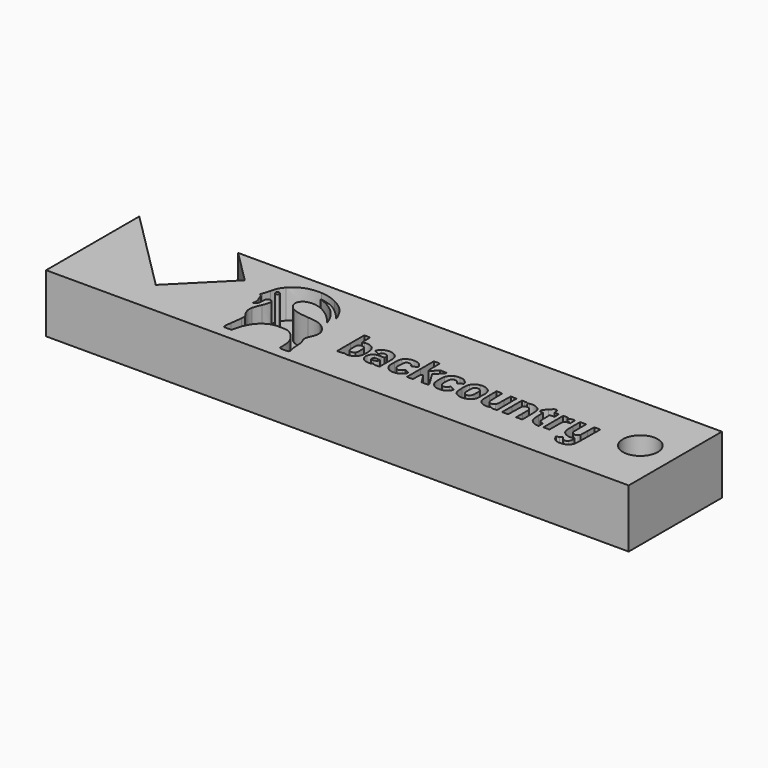
from build123d import *

# Parameters (mm, degrees)
F0_R     = 1.905
F1_DEPTH = 3.175
F3_DEPTH = 25.4


# Not quite as in the source:
# - ends of sketch curves that miss each other by under 0.0002 mm in the source are joined


with BuildPart() as f1:
    # F0 (on Top) → F1 (new body, symmetric)
    with BuildSketch(Plane.XY):
        Polygon((-31.75, -6.35), (31.75, -6.35), (31.75, 6.35), (-20.9736926547, 6.35), (-17.3815902063, 2.7578975516), (-22.7697438789, -2.6302561211), (-31.75, 6.35), align=None)
        with Locations((27.94, 0)):
            Circle(F0_R, mode=Mode.SUBTRACT)
    extrude(amount=F1_DEPTH, both=True)

    # F2 (on Top) → F3 (cut)
    with BuildSketch(Plane.XY):
        with BuildLine():
            add(Edge.make_bspline(
                [(-7.2094861414, -5.1238648126), (-7.2844689878, -5.0802139859), (-7.2989422964, -4.9953436696), (-7.2989422964, -4.5994253193)],
                knots=[0, 0, 0, 0, 1, 1, 1, 1], degree=3))
            add(Edge.make_bspline(
                [(-6.7301263581, -5.1775256832), (-6.9445733291, -5.1767519197), (-7.1602848509, -5.1525291904), (-7.2094861414, -5.1238648126)],
                knots=[0, 0, 0, 0, 1, 1, 1, 1], degree=3))
            add(Edge.make_bspline(
                [(-6.2994829734, -4.731018672), (-6.1786161943, -5.1344968151), (-6.2220690357, -5.1795470484), (-6.7301263581, -5.1775256832)],
                knots=[0, 0, 0, 0, 1, 1, 1, 1], degree=3))
            add(Edge.make_bspline(
                [(-6.4145096801, -3.7988983941), (-6.39840066, -4.1771751812), (-6.3514717779, -4.5574775093), (-6.2994829734, -4.731018672)],
                knots=[0, 0, 0, 0, 1, 1, 1, 1], degree=3))
            add(Edge.make_bspline(
                [(-6.5358053454, -2.9810219707), (-6.4648588427, -3.115930716), (-6.4350259592, -3.3170817273), (-6.4145096801, -3.7988983941)],
                knots=[0, 0, 0, 0, 1, 1, 1, 1], degree=3))
            add(Edge.make_bspline(
                [(-6.5204388926, -1.8308710912), (-6.7556023387, -2.2944279208), (-6.7591029433, -2.5564087833), (-6.5358053454, -2.9810219707)],
                knots=[0, 0, 0, 0, 1, 1, 1, 1], degree=3))
            add(Edge.make_bspline(
                [(-6.324628815, -0.7484458928), (-6.2534651672, -1.0310648715), (-6.3303639995, -1.4562130611), (-6.5204388926, -1.8308710912)],
                knots=[0, 0, 0, 0, 1, 1, 1, 1], degree=3))
            add(Edge.make_bspline(
                [(-7.3437616288, 0.4355162431), (-6.8349027857, 0.1658392581), (-6.4390507579, -0.294037896), (-6.324628815, -0.7484458928)],
                knots=[0, 0, 0, 0, 1, 1, 1, 1], degree=3))
            add(Edge.make_bspline(
                [(-8.9112722151, 0.7763364878), (-7.9235222683, 0.6866830845), (-7.7440808515, 0.6476672243), (-7.3437616288, 0.4355162431)],
                knots=[0, 0, 0, 0, 1, 1, 1, 1], degree=3))
            add(Edge.make_bspline(
                [(-10.647152276, 1.1281110135), (-10.2429696396, 0.9421016952), (-9.8416904589, 0.8607818482), (-8.9112722151, 0.7763364878)],
                knots=[0, 0, 0, 0, 1, 1, 1, 1], degree=3))
            add(Edge.make_bspline(
                [(-11.1241492556, 2.7289408409), (-11.6259189508, 2.2604417501), (-11.3904472275, 1.4701864746), (-10.647152276, 1.1281110135)],
                knots=[0, 0, 0, 0, 1, 1, 1, 1], degree=3))
            add(Edge.make_bspline(
                [(-8.9091506292, 2.683298617), (-9.760706155, 3.1170380384), (-10.6880443285, 3.1361554021), (-11.1241492556, 2.7289408409)],
                knots=[0, 0, 0, 0, 1, 1, 1, 1], degree=3))
            add(Edge.make_bspline(
                [(-7.1339415182, 1.1595366218), (-7.6226210992, 1.7916847381), (-8.2997509155, 2.3728951403), (-8.9091506292, 2.683298617)],
                knots=[0, 0, 0, 0, 1, 1, 1, 1], degree=3))
            Line((-7.1339415182, 1.1595366218), (-6.9956336173, 0.9806282421))
            Line((-6.9956336173, 0.9806282421), (-7.127209284, 1.3128911532))
            add(Edge.make_bspline(
                [(-10.0337398, 4.0116447856), (-8.5928247908, 3.5086741602), (-7.6501039523, 2.633343951), (-7.127209284, 1.3128911532)],
                knots=[0, 0, 0, 0, 1, 1, 1, 1], degree=3))
            add(Edge.make_bspline(
                [(-10.0546965102, 4.0691820888), (-10.1852513003, 4.0649715868), (-10.1849594809, 4.064364858), (-10.0337398, 4.0116447856)],
                knots=[0, 0, 0, 0, 1, 1, 1, 1], degree=3))
            add(Edge.make_bspline(
                [(-8.8503013669, 3.7439894114), (-9.1630163087, 3.8871481956), (-9.8592448202, 4.0751410506), (-10.0546965102, 4.0691820888)],
                knots=[0, 0, 0, 0, 1, 1, 1, 1], degree=3))
            add(Edge.make_bspline(
                [(-7.130290828, 2.3625743627), (-7.6390361859, 2.972923472), (-8.2660497056, 3.4765086867), (-8.8503013669, 3.7439894114)],
                knots=[0, 0, 0, 0, 1, 1, 1, 1], degree=3))
            add(Edge.make_bspline(
                [(-7.1493585727, 2.7186009034), (-6.8396981546, 2.0946875964), (-6.8350766982, 2.008395029), (-7.130290828, 2.3625743627)],
                knots=[0, 0, 0, 0, 1, 1, 1, 1], degree=3))
            add(Edge.make_bspline(
                [(-9.0113883754, 4.5370801004), (-8.1405818581, 4.1065971181), (-7.5538647159, 3.53360605), (-7.1493585727, 2.7186009034)],
                knots=[0, 0, 0, 0, 1, 1, 1, 1], degree=3))
            add(Edge.make_bspline(
                [(-10.8260663054, 5.0240893347), (-10.1563545479, 4.9803171623), (-9.6131202151, 4.8345413378), (-9.0113883754, 4.5370801004)],
                knots=[0, 0, 0, 0, 1, 1, 1, 1], degree=3))
            add(Edge.make_bspline(
                [(-13.8051989324, 3.9159186895), (-13.08035861, 4.7259186912), (-12.0617465513, 5.104821367), (-10.8260663054, 5.0240893347)],
                knots=[0, 0, 0, 0, 1, 1, 1, 1], degree=3))
            add(Edge.make_bspline(
                [(-14.4498235561, 2.5908043962), (-14.2578051655, 3.3284798592), (-14.1707658548, 3.5074034685), (-13.8051989324, 3.9159186895)],
                knots=[0, 0, 0, 0, 1, 1, 1, 1], degree=3))
            add(Edge.make_bspline(
                [(-14.688034648, 1.7996235521), (-14.6411774926, 1.9114476147), (-14.5339844663, 2.2674817702), (-14.4498235561, 2.5908043962)],
                knots=[0, 0, 0, 0, 1, 1, 1, 1], degree=3))
            Line((-14.688034648, 1.7996235521), (-14.7732262605, 1.5962915103))
            Line((-14.7732262605, 1.5962915103), (-14.6143239672, 1.4636357679))
            add(Edge.make_bspline(
                [(-14.4549225351, 1.2069010222), (-14.4552278646, 1.2827853645), (-14.5171373003, 1.3824942549), (-14.6143239672, 1.4636357679)],
                knots=[0, 0, 0, 0, 1, 1, 1, 1], degree=3))
            add(Edge.make_bspline(
                [(-14.3211822955, 0.8016854729), (-14.3944645815, 0.9563143806), (-14.4546476648, 1.1386631832), (-14.4549225351, 1.2069010222)],
                knots=[0, 0, 0, 0, 1, 1, 1, 1], degree=3))
            add(Edge.make_bspline(
                [(-14.2501196055, -0.0146468623), (-14.1499417898, 0.1725415242), (-14.1785020165, 0.5006207081), (-14.3211822955, 0.8016854729)],
                knots=[0, 0, 0, 0, 1, 1, 1, 1], degree=3))
            add(Edge.make_bspline(
                [(-14.209215271, -0.0723656929), (-14.3011165188, -0.1215701767), (-14.3046505302, -0.1165596279), (-14.2501196055, -0.0146468623)],
                knots=[0, 0, 0, 0, 1, 1, 1, 1], degree=3))
            add(Edge.make_bspline(
                [(-13.8350168319, 0.3838551214), (-13.8435589358, 0.2793442298), (-14.0716492006, 0.0012580317), (-14.209215271, -0.0723656929)],
                knots=[0, 0, 0, 0, 1, 1, 1, 1], degree=3))
            add(Edge.make_bspline(
                [(-13.8222340124, 0.7933261245), (-13.8254204444, 0.6151573646), (-13.831170613, 0.4308967519), (-13.8350168319, 0.3838551214)],
                knots=[0, 0, 0, 0, 1, 1, 1, 1], degree=3))
            add(Edge.make_bspline(
                [(-13.6957683784, 1.2150451906), (-13.7981544908, 1.1320790695), (-13.8173236844, 1.0681578486), (-13.8222340124, 0.7933261245)],
                knots=[0, 0, 0, 0, 1, 1, 1, 1], degree=3))
            add(Edge.make_bspline(
                [(-13.239967116, 1.2332895525), (-13.3921462637, 1.3398827278), (-13.5495113467, 1.3335899422), (-13.6957683784, 1.2150451906)],
                knots=[0, 0, 0, 0, 1, 1, 1, 1], degree=3))
            add(Edge.make_bspline(
                [(-13.4058914977, 0.1034508259), (-13.0922563913, 0.8460570051), (-13.0544697098, 1.1033611425), (-13.239967116, 1.2332895525)],
                knots=[0, 0, 0, 0, 1, 1, 1, 1], degree=3))
            add(Edge.make_bspline(
                [(-13.7437736516, -0.8304790761), (-13.7116843262, -0.6808415574), (-13.559634876, -0.2605678325), (-13.4058914977, 0.1034508259)],
                knots=[0, 0, 0, 0, 1, 1, 1, 1], degree=3))
            add(Edge.make_bspline(
                [(-13.4272002089, -2.0854137524), (-13.7319719152, -1.629746609), (-13.8309979286, -1.2371925334), (-13.7437736516, -0.8304790761)],
                knots=[0, 0, 0, 0, 1, 1, 1, 1], degree=3))
            Line((-13.4272002089, -2.0854137524), (-13.1835479625, -2.4497055617))
            Line((-13.1835479625, -2.4497055617), (-13.2267283901, -2.9070568077))
            add(Edge.make_bspline(
                [(-13.385989071, -4.1407085649), (-13.3221442439, -3.713739943), (-13.2504767901, -3.1585950556), (-13.2267283901, -2.9070568077)],
                knots=[0, 0, 0, 0, 1, 1, 1, 1], degree=3))
            add(Edge.make_bspline(
                [(-12.9747953999, -5.0768457809), (-13.5350716907, -5.0768457809), (-13.5282809944, -5.0922822409), (-13.385989071, -4.1407085649)],
                knots=[0, 0, 0, 0, 1, 1, 1, 1], degree=3))
            Line((-12.9747953999, -5.0768457809), (-12.5801614971, -5.0768457809))
            Line((-12.5801614971, -5.0768457809), (-12.4441709566, -4.5579439782))
            add(Edge.make_bspline(
                [(-11.1583272513, -2.4969370713), (-11.7594806107, -2.9076900656), (-12.1943534114, -3.6047149394), (-12.4441709566, -4.5579439782)],
                knots=[0, 0, 0, 0, 1, 1, 1, 1], degree=3))
            add(Edge.make_bspline(
                [(-9.5981627516, -2.0864606668), (-10.3550926451, -2.0864606668), (-10.6843422998, -2.1730870579), (-11.1583272513, -2.4969370713)],
                knots=[0, 0, 0, 0, 1, 1, 1, 1], degree=3))
            add(Edge.make_bspline(
                [(-8.6188156313, -2.2534928814), (-8.9472320778, -2.0918165844), (-8.9786503168, -2.0864606668), (-9.5981627516, -2.0864606668)],
                knots=[0, 0, 0, 0, 1, 1, 1, 1], degree=3))
            add(Edge.make_bspline(
                [(-8.0064783182, -2.7162228894), (-8.1877190423, -2.5199419214), (-8.3935885373, -2.3643724611), (-8.6188156313, -2.2534928814)],
                knots=[0, 0, 0, 0, 1, 1, 1, 1], degree=3))
            add(Edge.make_bspline(
                [(-7.2989422964, -4.5994253193), (-7.2989422964, -3.7967249783), (-7.4980166736, -3.266861034), (-8.0064783182, -2.7162228894)],
                knots=[0, 0, 0, 0, 1, 1, 1, 1], degree=3))
        make_face()
        with BuildLine():
            add(Edge.make_bspline(
                [(-13.5352993982, 2.5396888392), (-13.4147126478, 2.765009276), (-13.7303347298, 2.9658721525), (-13.894380217, 2.768210692)],
                knots=[0, 0, 0, 0, 1, 1, 1, 1], degree=3))
            add(Edge.make_bspline(
                [(-13.901734901, 2.5637366734), (-13.8297500813, 2.4057474211), (-13.6145418743, 2.3916256222), (-13.5352993982, 2.5396888392)],
                knots=[0, 0, 0, 0, 1, 1, 1, 1], degree=3))
            add(Edge.make_bspline(
                [(-13.894380217, 2.768210692), (-13.9439963922, 2.7084393001), (-13.9457288857, 2.660293767), (-13.901734901, 2.5637366734)],
                knots=[0, 0, 0, 0, 1, 1, 1, 1], degree=3))
        make_face(mode=Mode.SUBTRACT)
        with BuildLine():
            add(Edge.make_bspline(
                [(21.9914919475, -3.8684142939), (21.6825117045, -3.7441034072), (21.5586726907, -3.6547914425), (21.4241410016, -3.4592579546)],
                knots=[0, 0, 0, 0, 1, 1, 1, 1], degree=3))
            add(Edge.make_bspline(
                [(22.4177177564, -3.8810792066), (22.2254542179, -3.8910553523), (22.0336419186, -3.8852889716), (21.9914919475, -3.8684142939)],
                knots=[0, 0, 0, 0, 1, 1, 1, 1], degree=3))
            add(Edge.make_bspline(
                [(23.2904181521, -3.3643208517), (23.1198290816, -3.6909470796), (22.8353363669, -3.8594094057), (22.4177177564, -3.8810792066)],
                knots=[0, 0, 0, 0, 1, 1, 1, 1], degree=3))
            add(Edge.make_bspline(
                [(23.411965352, -1.4857457735), (23.3980007622, -3.0686346033), (23.3913685032, -3.1709873087), (23.2904181521, -3.3643208517)],
                knots=[0, 0, 0, 0, 1, 1, 1, 1], degree=3))
            Line((23.411965352, -1.4857457735), (23.4267589741, 0.1883626553))
            Line((23.4267589741, 0.1883626553), (23.0957318739, 0.1883626553))
            Line((23.0957318739, 0.1883626553), (22.7647158275, 0.1883626553))
            Line((22.7647158275, 0.1883626553), (22.7487062912, -0.7362968225))
            Line((22.7487062912, -0.7362968225), (22.7326967549, -1.6609484399))
            Line((22.7326967549, -1.6609484399), (22.5892758737, -1.7842047974))
            add(Edge.make_bspline(
                [(22.0386767857, -1.7580705037), (22.2214028902, -1.9407985733), (22.397362371, -1.9491586585), (22.5892758737, -1.7842047974)],
                knots=[0, 0, 0, 0, 1, 1, 1, 1], degree=3))
            Line((22.0386767857, -1.7580705037), (21.8892539557, -1.6086496388))
            Line((21.8892539557, -1.6086496388), (21.8892539557, -0.710154914))
            Line((21.8892539557, -0.710154914), (21.8892539557, 0.1883361262))
            Line((21.8892539557, 0.1883361262), (21.5569905533, 0.1883361262))
            Line((21.5569905533, 0.1883361262), (21.2247273966, 0.1883361262))
            Line((21.2247273966, 0.1883361262), (21.2247273966, -0.772072947))
            add(Edge.make_bspline(
                [(21.3397418213, -1.9601470835), (21.2326251888, -1.7481135178), (21.2247273966, -1.6665129052), (21.2247273966, -0.772072947)],
                knots=[0, 0, 0, 0, 1, 1, 1, 1], degree=3))
            add(Edge.make_bspline(
                [(22.6688003436, -2.4437957276), (22.1901391582, -2.6367652333), (21.567008949, -2.4099994553), (21.3397418213, -1.9601470835)],
                knots=[0, 0, 0, 0, 1, 1, 1, 1], degree=3))
            add(Edge.make_bspline(
                [(22.7582564985, -2.698277716), (22.7582564985, -2.4419070077), (22.7477556674, -2.4119716926), (22.6688003436, -2.4437957276)],
                knots=[0, 0, 0, 0, 1, 1, 1, 1], degree=3))
            add(Edge.make_bspline(
                [(22.6088373531, -3.1382492501), (22.7389310784, -3.0081538053), (22.7582564985, -2.9512536903), (22.7582564985, -2.698277716)],
                knots=[0, 0, 0, 0, 1, 1, 1, 1], degree=3))
            add(Edge.make_bspline(
                [(22.0069728682, -3.1016079843), (22.2270771562, -3.3349812117), (22.401494514, -3.3456134598), (22.6088373531, -3.1382492501)],
                knots=[0, 0, 0, 0, 1, 1, 1, 1], degree=3))
            Line((22.0069728682, -3.1016079843), (21.8314683112, -2.9155190789))
            Line((21.8314683112, -2.9155190789), (21.575857365, -3.0352362665))
            add(Edge.make_bspline(
                [(21.2952926671, -3.1953426832), (21.3089809128, -3.1731150356), (21.4352758275, -3.1010842815), (21.575857365, -3.0352362665)],
                knots=[0, 0, 0, 0, 1, 1, 1, 1], degree=3))
            add(Edge.make_bspline(
                [(21.4241410016, -3.4592579546), (21.3395482576, -3.3363125763), (21.2815712602, -3.2175472407), (21.2952926671, -3.1953426832)],
                knots=[0, 0, 0, 0, 1, 1, 1, 1], degree=3))
        make_face()
        with BuildLine():
            add(Edge.make_bspline(
                [(2.650465598, -2.4971684634), (2.3900189981, -2.4043210134), (2.1786395696, -2.1954625803), (2.0777464525, -1.9312665432)],
                knots=[0, 0, 0, 0, 1, 1, 1, 1], degree=3))
            add(Edge.make_bspline(
                [(4.0037628162, -2.1471347828), (3.7299667071, -2.5250969061), (3.1497626888, -2.675174119), (2.650465598, -2.4971684634)],
                knots=[0, 0, 0, 0, 1, 1, 1, 1], degree=3))
            add(Edge.make_bspline(
                [(4.1514170438, -1.8992946334), (4.1514170438, -1.9234945183), (4.0849748276, -2.0350265157), (4.0037628162, -2.1471347828)],
                knots=[0, 0, 0, 0, 1, 1, 1, 1], degree=3))
            add(Edge.make_bspline(
                [(3.869682612, -1.7171204802), (4.0246342896, -1.7931146233), (4.1514170438, -1.8750986787), (4.1514170438, -1.8992946334)],
                knots=[0, 0, 0, 0, 1, 1, 1, 1], degree=3))
            Line((3.869682612, -1.7171204802), (3.5879533385, -1.5789457158))
            Line((3.5879533385, -1.5789457158), (3.4314617486, -1.7687936383))
            add(Edge.make_bspline(
                [(2.8326178893, -1.8549913889), (3.0155847202, -2.0254490425), (3.2474138595, -1.9920811649), (3.4314617486, -1.7687936383)],
                knots=[0, 0, 0, 0, 1, 1, 1, 1], degree=3))
            add(Edge.make_bspline(
                [(2.6764994253, -1.0704221702), (2.6551860469, -1.5772237849), (2.6827190104, -1.7153147863), (2.8326178893, -1.8549913889)],
                knots=[0, 0, 0, 0, 1, 1, 1, 1], degree=3))
            add(Edge.make_bspline(
                [(3.0161885014, -0.4097501818), (2.7683301746, -0.4571445502), (2.696375323, -0.5970638443), (2.6764994253, -1.0704221702)],
                knots=[0, 0, 0, 0, 1, 1, 1, 1], degree=3))
            add(Edge.make_bspline(
                [(3.4373959009, -0.5669961297), (3.4343708539, -0.4912938061), (3.1481024133, -0.3845299116), (3.0161885014, -0.4097501818)],
                knots=[0, 0, 0, 0, 1, 1, 1, 1], degree=3))
            add(Edge.make_bspline(
                [(3.509320539, -0.6967498903), (3.4706819806, -0.6457330803), (3.4382890452, -0.5873610951), (3.4373959009, -0.5669961297)],
                knots=[0, 0, 0, 0, 1, 1, 1, 1], degree=3))
            add(Edge.make_bspline(
                [(3.8527408748, -0.6522533278), (3.5918165066, -0.783338453), (3.5764758459, -0.7853264112), (3.509320539, -0.6967498903)],
                knots=[0, 0, 0, 0, 1, 1, 1, 1], degree=3))
            add(Edge.make_bspline(
                [(4.1424082254, -0.5003858963), (4.1332891149, -0.5084661985), (4.0029539262, -0.5767900112), (3.8527408748, -0.6522533278)],
                knots=[0, 0, 0, 0, 1, 1, 1, 1], degree=3))
            add(Edge.make_bspline(
                [(3.8228549332, -0.0262690365), (3.9856992447, -0.169249241), (4.1840313003, -0.4635132383), (4.1424082254, -0.5003858963)],
                knots=[0, 0, 0, 0, 1, 1, 1, 1], degree=3))
            add(Edge.make_bspline(
                [(2.1672345405, -0.235628328), (2.4917632551, 0.2541841412), (3.3760794383, 0.3660042735), (3.8228549332, -0.0262690365)],
                knots=[0, 0, 0, 0, 1, 1, 1, 1], degree=3))
            add(Edge.make_bspline(
                [(2.0129394565, -1.0797569519), (2.0288183128, -0.4888091654), (2.0399882651, -0.4277179539), (2.1672345405, -0.235628328)],
                knots=[0, 0, 0, 0, 1, 1, 1, 1], degree=3))
            add(Edge.make_bspline(
                [(2.0777464525, -1.9312665432), (2.0143462324, -1.7652583986), (1.9997051522, -1.5729187119), (2.0129394565, -1.0797569519)],
                knots=[0, 0, 0, 0, 1, 1, 1, 1], degree=3))
        make_face()
        with BuildLine():
            add(Edge.make_bspline(
                [(7.6298325146, -2.5053222118), (7.368764693, -2.4220944849), (7.0921975278, -2.120153525), (7.022120588, -1.8418509188)],
                knots=[0, 0, 0, 0, 1, 1, 1, 1], degree=3))
            Line((7.6298325146, -2.5053222118), (7.6300425361, -2.505352671))
            add(Edge.make_bspline(
                [(8.5769264681, -2.475273657), (8.3441673387, -2.5809906372), (7.9105519652, -2.5947557679), (7.6300425361, -2.505352671)],
                knots=[0, 0, 0, 0, 1, 1, 1, 1], degree=3))
            add(Edge.make_bspline(
                [(9.1100458691, -1.9208573356), (9.1100458691, -2.0432942407), (8.7859514446, -2.3803402387), (8.5769264681, -2.475273657)],
                knots=[0, 0, 0, 0, 1, 1, 1, 1], degree=3))
            add(Edge.make_bspline(
                [(8.8251404805, -1.7155412657), (8.9818369335, -1.7923929352), (9.1100458691, -1.8847849702), (9.1100458691, -1.9208573356)],
                knots=[0, 0, 0, 0, 1, 1, 1, 1], degree=3))
            add(Edge.make_bspline(
                [(8.4871055389, -1.6707413387), (8.5378199671, -1.580090149), (8.5530945508, -1.5821117598), (8.8251404805, -1.7155412657)],
                knots=[0, 0, 0, 0, 1, 1, 1, 1], degree=3))
            add(Edge.make_bspline(
                [(7.801436812, -1.8393932983), (8.0393081849, -2.0439999622), (8.3163580311, -1.9758606245), (8.4871055389, -1.6707413387)],
                knots=[0, 0, 0, 0, 1, 1, 1, 1], degree=3))
            add(Edge.make_bspline(
                [(7.6390513546, -1.3093662496), (7.6603649786, -1.6779402874), (7.6770856404, -1.7324282253), (7.801436812, -1.8393932983)],
                knots=[0, 0, 0, 0, 1, 1, 1, 1], degree=3))
            add(Edge.make_bspline(
                [(7.9119282817, -0.446029621), (7.6813376554, -0.5423779213), (7.6080713359, -0.7741810228), (7.6390513546, -1.3093662496)],
                knots=[0, 0, 0, 0, 1, 1, 1, 1], degree=3))
            add(Edge.make_bspline(
                [(8.4417924717, -0.624323657), (8.2904276179, -0.4117555804), (8.1262128852, -0.356493879), (7.9119282817, -0.446029621)],
                knots=[0, 0, 0, 0, 1, 1, 1, 1], degree=3))
            Line((8.4417924717, -0.624323657), (8.5523227524, -0.7795519244))
            Line((8.5523227524, -0.7795519244), (8.8311851705, -0.642788603))
            add(Edge.make_bspline(
                [(9.1100458691, -0.4588085103), (9.1100458691, -0.4847534162), (8.9845541946, -0.5675677322), (8.8311851705, -0.642788603)],
                knots=[0, 0, 0, 0, 1, 1, 1, 1], degree=3))
            add(Edge.make_bspline(
                [(8.6710512422, 0.0658736746), (8.8737586235, -0.0529221203), (9.1100458691, -0.335328621), (9.1100458691, -0.4588085103)],
                knots=[0, 0, 0, 0, 1, 1, 1, 1], degree=3))
            add(Edge.make_bspline(
                [(8.1004244515, 0.1982751804), (8.3790768481, 0.1981309902), (8.4888132228, 0.172671713), (8.6710512422, 0.0658736746)],
                knots=[0, 0, 0, 0, 1, 1, 1, 1], degree=3))
            add(Edge.make_bspline(
                [(7.5711461111, 0.119124819), (7.6774079191, 0.1648883886), (7.9014972122, 0.198377612), (8.1004244515, 0.1982751804)],
                knots=[0, 0, 0, 0, 1, 1, 1, 1], degree=3))
            add(Edge.make_bspline(
                [(7.0172935317, -0.5131446431), (7.0856998791, -0.2668141923), (7.3345606595, 0.0172803412), (7.5711461111, 0.119124819)],
                knots=[0, 0, 0, 0, 1, 1, 1, 1], degree=3))
            add(Edge.make_bspline(
                [(7.022120588, -1.8418509188), (6.9483826412, -1.5490325083), (6.9454366901, -0.7711350965), (7.0172935317, -0.5131446431)],
                knots=[0, 0, 0, 0, 1, 1, 1, 1], degree=3))
        make_face()
        with BuildLine():
            add(Edge.make_bspline(
                [(10.1145621667, -2.4974705997), (9.6278484363, -2.3239331216), (9.4703286006, -2.004801592), (9.4687756694, -1.1891138141)],
                knots=[0, 0, 0, 0, 1, 1, 1, 1], degree=3))
            add(Edge.make_bspline(
                [(11.4838455854, -2.1456427702), (11.1751748477, -2.5333872298), (10.617306067, -2.6767241025), (10.1145621667, -2.4974705997)],
                knots=[0, 0, 0, 0, 1, 1, 1, 1], degree=3))
            add(Edge.make_bspline(
                [(11.6579350148, -1.2647630797), (11.6404147973, -1.939708672), (11.6379498077, -1.9520321462), (11.4838455854, -2.1456427702)],
                knots=[0, 0, 0, 0, 1, 1, 1, 1], degree=3))
            add(Edge.make_bspline(
                [(11.5622850669, -0.3459375334), (11.6655805356, -0.5593137631), (11.6741214114, -0.6413543156), (11.6579350148, -1.2647630797)],
                knots=[0, 0, 0, 0, 1, 1, 1, 1], degree=3))
            add(Edge.make_bspline(
                [(10.3297514594, 0.1870138503), (10.8587645095, 0.2873370844), (11.360811777, 0.0702548958), (11.5622850669, -0.3459375334)],
                knots=[0, 0, 0, 0, 1, 1, 1, 1], degree=3))
            add(Edge.make_bspline(
                [(9.5945802882, -0.3456719974), (9.7473600239, -0.0413073153), (9.9677111793, 0.1183549857), (10.3297514594, 0.1870138503)],
                knots=[0, 0, 0, 0, 1, 1, 1, 1], degree=3))
            add(Edge.make_bspline(
                [(9.4687756694, -1.1891138141), (9.4674858179, -0.6609076889), (9.4811006174, -0.5718082021), (9.5945802882, -0.3456719974)],
                knots=[0, 0, 0, 0, 1, 1, 1, 1], degree=3))
        make_face()
        with BuildLine():
            add(Edge.make_bspline(
                [(10.8011503212, -1.8930991209), (10.9558423582, -1.7743261705), (11.0011846566, -1.6051964426), (11.0011846566, -1.1469461571)],
                knots=[0, 0, 0, 0, 1, 1, 1, 1], degree=3))
            add(Edge.make_bspline(
                [(10.3011701077, -1.8352432237), (10.4557680649, -1.9682173145), (10.6708723665, -1.993103761), (10.8011503212, -1.8930991209)],
                knots=[0, 0, 0, 0, 1, 1, 1, 1], degree=3))
            add(Edge.make_bspline(
                [(10.1577418573, -1.1721283532), (10.1577418573, -1.7001448449), (10.1607632197, -1.7145508483), (10.3011701077, -1.8352432237)],
                knots=[0, 0, 0, 0, 1, 1, 1, 1], degree=3))
            add(Edge.make_bspline(
                [(10.2716214288, -0.5185076842), (10.168242934, -0.6218883898), (10.1577418573, -0.6821488493), (10.1577418573, -1.1721283532)],
                knots=[0, 0, 0, 0, 1, 1, 1, 1], degree=3))
            add(Edge.make_bspline(
                [(10.8800169693, -0.5455144885), (10.7233133927, -0.3633327205), (10.4394121773, -0.3507356043), (10.2716214288, -0.5185076842)],
                knots=[0, 0, 0, 0, 1, 1, 1, 1], degree=3))
            add(Edge.make_bspline(
                [(11.0011846566, -1.1469461571), (11.0011846566, -0.7360865554), (10.988085945, -0.6711793386), (10.8800169693, -0.5455144885)],
                knots=[0, 0, 0, 0, 1, 1, 1, 1], degree=3))
        make_face(mode=Mode.SUBTRACT)
        with BuildLine():
            add(Edge.make_bspline(
                [(18.4254680201, -2.5037972835), (18.1741311963, -2.412645481), (17.9010867432, -2.1727026325), (17.8123488373, -1.9650082837)],
                knots=[0, 0, 0, 0, 1, 1, 1, 1], degree=3))
            add(Edge.make_bspline(
                [(18.7582841107, -2.5682090459), (18.6669136893, -2.5659319703), (18.5171388583, -2.5371054707), (18.4254680201, -2.5037972835)],
                knots=[0, 0, 0, 0, 1, 1, 1, 1], degree=3))
            Line((18.7582841107, -2.5682090459), (18.9244202334, -2.5720022068))
            Line((18.9244202334, -2.5720022068), (18.9244202334, -2.2904456177))
            add(Edge.make_bspline(
                [(18.7184573954, -1.9264724025), (18.9240942702, -2.008751962), (18.9244202334, -2.0093324075), (18.9244202334, -2.2904456177)],
                knots=[0, 0, 0, 0, 1, 1, 1, 1], degree=3))
            add(Edge.make_bspline(
                [(18.4628702762, -1.7513343393), (18.490143599, -1.8023513949), (18.6051801313, -1.8811487728), (18.7184573954, -1.9264724025)],
                knots=[0, 0, 0, 0, 1, 1, 1, 1], degree=3))
            add(Edge.make_bspline(
                [(18.413242556, -1.0418376252), (18.413242556, -1.3810609693), (18.435582215, -1.7003361978), (18.4628702762, -1.7513343393)],
                knots=[0, 0, 0, 0, 1, 1, 1, 1], degree=3))
            Line((18.413242556, -1.0418376252), (18.413242556, -0.425059155))
            Line((18.413242556, -0.425059155), (18.6713811298, -0.425059155))
            Line((18.6713811298, -0.425059155), (18.9295216688, -0.425059155))
            Line((18.9295216688, -0.425059155), (18.9141937813, -0.1311368419))
            Line((18.9141937813, -0.1311368419), (18.8988658939, 0.1627891559))
            Line((18.8988658939, 0.1627891559), (18.658744957, 0.1782644268))
            Line((18.658744957, 0.1782644268), (18.4186277047, 0.1937011325))
            Line((18.4186277047, 0.1937011325), (18.4031524337, 0.4338220694))
            add(Edge.make_bspline(
                [(18.2148183858, 0.690458805), (18.3817651179, 0.6745283645), (18.3882205166, 0.6656895284), (18.4031524337, 0.4338220694)],
                knots=[0, 0, 0, 0, 1, 1, 1, 1], degree=3))
            add(Edge.make_bspline(
                [(17.6663765015, 0.307076161), (18.0088314752, 0.6717094088), (18.0572044702, 0.7055209108), (18.2148183858, 0.690458805)],
                knots=[0, 0, 0, 0, 1, 1, 1, 1], degree=3))
            add(Edge.make_bspline(
                [(17.2897268286, -0.2589620889), (17.2904637462, -0.1235755753), (17.360305118, -0.0188104471), (17.6663765015, 0.307076161)],
                knots=[0, 0, 0, 0, 1, 1, 1, 1], degree=3))
            add(Edge.make_bspline(
                [(17.4864582989, -0.4250876491), (17.2971532392, -0.4250876491), (17.2886988284, -0.4179562513), (17.2897268286, -0.2589620889)],
                knots=[0, 0, 0, 0, 1, 1, 1, 1], degree=3))
            Line((17.4864582989, -0.4250876491), (17.6842614932, -0.4250876491))
            Line((17.6842614932, -0.4250876491), (17.7087254403, -1.10240366))
            add(Edge.make_bspline(
                [(17.8123488373, -1.9650082837), (17.7598839841, -1.8422412395), (17.7249339443, -1.5511523748), (17.7087254403, -1.10240366)],
                knots=[0, 0, 0, 0, 1, 1, 1, 1], degree=3))
        make_face()
        with BuildLine():
            add(Edge.make_bspline(
                [(-2.2087901256, 0.1154033848), (-1.8307363789, 0.2291807704), (-1.3859264891, 0.0817586719), (-1.1418829394, -0.2381957491)],
                knots=[0, 0, 0, 0, 1, 1, 1, 1], degree=3))
            Line((-2.2087901256, 0.1154033848), (-2.4395259247, 0.0459631419))
            Line((-2.4395259247, 0.0459631419), (-2.4539235764, 0.615544492))
            Line((-2.4539235764, 0.615544492), (-2.4683209825, 1.185129281))
            Line((-2.4683209825, 1.185129281), (-2.7878067239, 1.2003409811))
            Line((-2.7878067239, 1.2003409811), (-3.1072924652, 1.2155529269))
            Line((-3.1072924652, 1.2155529269), (-3.1072924652, -0.6526817226))
            Line((-3.1072924652, -0.6526817226), (-3.1073017995, -2.5208665074))
            Line((-3.1073017995, -2.5208665074), (-2.8363777041, -2.5208665074))
            add(Edge.make_bspline(
                [(-2.5088185385, -2.464235613), (-2.5399673113, -2.4953770166), (-2.6873700044, -2.5208665074), (-2.8363777041, -2.5208665074)],
                knots=[0, 0, 0, 0, 1, 1, 1, 1], degree=3))
            add(Edge.make_bspline(
                [(-2.262178091, -2.4703429409), (-2.4011890113, -2.4244543409), (-2.4673836232, -2.4228269811), (-2.5088185385, -2.464235613)],
                knots=[0, 0, 0, 0, 1, 1, 1, 1], degree=3))
            add(Edge.make_bspline(
                [(-1.0734903478, -2.0181845081), (-1.2834661937, -2.3917882546), (-1.8487127485, -2.6067952831), (-2.262178091, -2.4703429409)],
                knots=[0, 0, 0, 0, 1, 1, 1, 1], degree=3))
            add(Edge.make_bspline(
                [(-1.1418829394, -0.2381957491), (-0.8746237813, -0.5885895368), (-0.8359356038, -1.5955172747), (-1.0734903478, -2.0181845081)],
                knots=[0, 0, 0, 0, 1, 1, 1, 1], degree=3))
        make_face()
        with BuildLine():
            add(Edge.make_bspline(
                [(-1.7143353208, -1.7483336105), (-1.6438199149, -1.663402867), (-1.6248791658, -1.5436702041), (-1.6248791658, -1.1828340474)],
                knots=[0, 0, 0, 0, 1, 1, 1, 1], degree=3))
            add(Edge.make_bspline(
                [(-2.2127326351, -1.8505799542), (-2.0727828817, -1.9300110812), (-1.8225504518, -1.8786491481), (-1.7143353208, -1.7483336105)],
                knots=[0, 0, 0, 0, 1, 1, 1, 1], degree=3))
            add(Edge.make_bspline(
                [(-2.4427624671, -1.1654425448), (-2.4427624671, -1.6448998469), (-2.4116021492, -1.7377131531), (-2.2127326351, -1.8505799542)],
                knots=[0, 0, 0, 0, 1, 1, 1, 1], degree=3))
            add(Edge.make_bspline(
                [(-2.3277477967, -0.5949739458), (-2.4310724965, -0.6879766399), (-2.4427624671, -0.7459614977), (-2.4427624671, -1.1654425448)],
                knots=[0, 0, 0, 0, 1, 1, 1, 1], degree=3))
            add(Edge.make_bspline(
                [(-1.8808290942, -0.4837455584), (-2.0589944152, -0.4216376463), (-2.1642930718, -0.4478249981), (-2.3277477967, -0.5949739458)],
                knots=[0, 0, 0, 0, 1, 1, 1, 1], degree=3))
            add(Edge.make_bspline(
                [(-1.6248791658, -1.1828340474), (-1.6248791658, -0.6615198218), (-1.6620399586, -0.5600094133), (-1.8808290942, -0.4837455584)],
                knots=[0, 0, 0, 0, 1, 1, 1, 1], degree=3))
        make_face(mode=Mode.SUBTRACT)
        with BuildLine():
            add(Edge.make_bspline(
                [(-0.1917521482, -2.4059068602), (-0.744070465, -2.1226922064), (-0.7445536374, -1.3031314349), (-0.1923601052, -1.0258077009)],
                knots=[0, 0, 0, 0, 1, 1, 1, 1], degree=3))
            Line((-0.1917521482, -2.4059068602), (-0.1915448287, -2.4061163905))
            add(Edge.make_bspline(
                [(0.6853751576, -2.4647991093), (0.5029032897, -2.5624522451), (0.054864718, -2.5324680478), (-0.1915448286, -2.4061163905)],
                knots=[0, 0, 0, 0, 1, 1, 1, 1], degree=3))
            add(Edge.make_bspline(
                [(0.9019110446, -2.4678334906), (0.8200119803, -2.4240003997), (0.7628485401, -2.4231546638), (0.6853751576, -2.4647991093)],
                knots=[0, 0, 0, 0, 1, 1, 1, 1], degree=3))
            add(Edge.make_bspline(
                [(1.2661242493, -2.5113629715), (1.1270077041, -2.5201617685), (0.963107144, -2.5005523894), (0.9019110446, -2.4678334906)],
                knots=[0, 0, 0, 0, 1, 1, 1, 1], degree=3))
            Line((1.2661242493, -2.5113629715), (1.519066571, -2.4953554004))
            Line((1.519066571, -2.4953554004), (1.519066571, -1.4985627368))
            add(Edge.make_bspline(
                [(1.3835058992, -0.2711885356), (1.5176595496, -0.4993691955), (1.519066571, -0.5121291706), (1.519066571, -1.4985627368)],
                knots=[0, 0, 0, 0, 1, 1, 1, 1], degree=3))
            add(Edge.make_bspline(
                [(-0.2828865103, 0.0004417725), (0.2531365919, 0.4007450286), (1.0663972087, 0.2681843487), (1.3835058992, -0.2711885356)],
                knots=[0, 0, 0, 0, 1, 1, 1, 1], degree=3))
            add(Edge.make_bspline(
                [(-0.5822025694, -0.4674009703), (-0.6257934601, -0.3968344715), (-0.4528548505, -0.1264937693), (-0.2828865103, 0.0004417725)],
                knots=[0, 0, 0, 0, 1, 1, 1, 1], degree=3))
            add(Edge.make_bspline(
                [(-0.3084010563, -0.6235737205), (-0.4456276533, -0.5592997616), (-0.5688415152, -0.4890216433), (-0.5822025694, -0.4674009703)],
                knots=[0, 0, 0, 0, 1, 1, 1, 1], degree=3))
            Line((-0.3084010563, -0.6235737205), (-0.0588881037, -0.7404348609))
            Line((-0.0588881037, -0.7404348609), (0.1305206158, -0.5510273696))
            add(Edge.make_bspline(
                [(0.4816451802, -0.39395951), (0.3422203578, -0.3660801952), (0.2938237813, -0.3877379598), (0.1305206158, -0.5510273696)],
                knots=[0, 0, 0, 0, 1, 1, 1, 1], degree=3))
            add(Edge.make_bspline(
                [(0.8289775663, -0.7652797943), (0.8289775663, -0.5649062312), (0.7122119795, -0.4400755719), (0.4816451802, -0.39395951)],
                knots=[0, 0, 0, 0, 1, 1, 1, 1], degree=3))
            Line((0.8289775663, -0.7652797943), (0.8289775663, -0.9362682742))
            Line((0.8289775663, -0.9362682742), (0.4072506398, -0.9363478613))
            add(Edge.make_bspline(
                [(-0.1923601052, -1.0258077009), (-0.0660425917, -0.9623379649), (0.1077957944, -0.936401165), (0.4072506398, -0.9363478613)],
                knots=[0, 0, 0, 0, 1, 1, 1, 1], degree=3))
        make_face()
        with BuildLine():
            add(Edge.make_bspline(
                [(0.7360642849, -1.7550776354), (0.9134646854, -1.5359929958), (0.8644761185, -1.4926379188), (0.4581691941, -1.5091036071)],
                knots=[0, 0, 0, 0, 1, 1, 1, 1], degree=3))
            add(Edge.make_bspline(
                [(0.3791016131, -1.8949554165), (0.5710770169, -1.8764831014), (0.6687156599, -1.8382638492), (0.7360642849, -1.7550776354)],
                knots=[0, 0, 0, 0, 1, 1, 1, 1], degree=3))
            add(Edge.make_bspline(
                [(0.0707411178, -1.6428517071), (0.0374756718, -1.877435199), (0.0925968676, -1.9224815021), (0.3791016131, -1.8949554165)],
                knots=[0, 0, 0, 0, 1, 1, 1, 1], degree=3))
            add(Edge.make_bspline(
                [(0.4581691941, -1.5091036071), (0.1144769356, -1.5230627928), (0.0863421561, -1.53277242), (0.0707411178, -1.6428517071)],
                knots=[0, 0, 0, 0, 1, 1, 1, 1], degree=3))
        make_face(mode=Mode.SUBTRACT)
        with BuildLine():
            add(Edge.make_bspline(
                [(5.1737687141, 0.3446869649), (5.1737687141, -0.2235814436), (5.1919337345, -0.4813898783), (5.2337206508, -0.5072360373)],
                knots=[0, 0, 0, 0, 1, 1, 1, 1], degree=3))
            Line((5.1737687141, 0.3446869649), (5.1737687141, 1.1595518514))
            Line((5.1737687141, 1.1595518514), (4.8415055573, 1.1595518514))
            Line((4.8415055573, 1.1595518514), (4.5092421549, 1.1595518514))
            Line((4.5092421549, 1.1595518514), (4.5092421549, -0.6806823832))
            Line((4.5092421549, -0.6806823832), (4.5092239776, -2.5207508113))
            Line((4.5092239776, -2.5207508113), (4.8414871344, -2.5207508113))
            Line((4.8414871344, -2.5207508113), (5.1737502911, -2.5207508113))
            Line((5.1737502911, -2.5207508113), (5.1737502911, -2.0174957357))
            add(Edge.make_bspline(
                [(5.2723977745, -1.424973893), (5.1876726309, -1.5016435439), (5.1737502911, -1.5852696976), (5.1737502911, -2.0174957357)],
                knots=[0, 0, 0, 0, 1, 1, 1, 1], degree=3))
            add(Edge.make_bspline(
                [(5.8596125818, -2.1245895238), (5.3148110707, -1.2430689605), (5.3832707219, -1.3246278145), (5.2723977745, -1.424973893)],
                knots=[0, 0, 0, 0, 1, 1, 1, 1], degree=3))
            Line((5.8596125818, -2.1245895238), (6.1044515112, -2.5207508113))
            Line((6.1044515112, -2.5207508113), (6.5099018916, -2.5207508113))
            add(Edge.make_bspline(
                [(6.3413172371, -1.5647416278), (7.0085114382, -2.6392810702), (6.9876087686, -2.5207508113), (6.5099018916, -2.5207508113)],
                knots=[0, 0, 0, 0, 1, 1, 1, 1], degree=3))
            add(Edge.make_bspline(
                [(5.8894024784, -0.7958491042), (5.8894024784, -0.818417699), (6.092763997, -1.1644307569), (6.3413172371, -1.5647416278)],
                knots=[0, 0, 0, 0, 1, 1, 1, 1], degree=3))
            add(Edge.make_bspline(
                [(6.2983419183, -0.3482460508), (6.073425558, -0.5718484869), (5.8894024784, -0.7732687188), (5.8894024784, -0.7958491042)],
                knots=[0, 0, 0, 0, 1, 1, 1, 1], degree=3))
            add(Edge.make_bspline(
                [(6.7072816039, 0.1233937831), (6.7072816039, 0.0875869537), (6.5232585243, -0.1246472993), (6.2983419183, -0.3482460508)],
                knots=[0, 0, 0, 0, 1, 1, 1, 1], degree=3))
            add(Edge.make_bspline(
                [(6.3366800599, 0.1897802392), (6.602047796, 0.1886564398), (6.7072816039, 0.1699804897), (6.7072816039, 0.1233937831)],
                knots=[0, 0, 0, 0, 1, 1, 1, 1], degree=3))
            Line((6.3366800599, 0.1897802392), (5.9660767965, 0.1909040387))
            Line((5.9660767965, 0.1909040387), (5.6298839035, -0.1766953027))
            add(Edge.make_bspline(
                [(5.2337206508, -0.5072360373), (5.2706090297, -0.5300704137), (5.4229242615, -0.4029946119), (5.6298839035, -0.1766953027)],
                knots=[0, 0, 0, 0, 1, 1, 1, 1], degree=3))
        make_face()
        with BuildLine():
            add(Edge.make_bspline(
                [(12.796793368, -2.4443570133), (12.6738460246, -2.4060203455), (12.508133384, -2.3122515028), (12.4285519257, -2.2360028775)],
                knots=[0, 0, 0, 0, 1, 1, 1, 1], degree=3))
            Line((12.7967933681, -2.4443570133), (12.7968781136, -2.4443017444))
            add(Edge.make_bspline(
                [(13.4709367027, -2.4589054875), (13.2140341855, -2.5358711336), (13.0812693793, -2.5329996111), (12.7968781136, -2.4443017444)],
                knots=[0, 0, 0, 0, 1, 1, 1, 1], degree=3))
            add(Edge.make_bspline(
                [(13.6983789712, -2.4589054875), (13.6821852055, -2.4103654577), (13.6329112057, -2.4103654577), (13.4709367027, -2.4589054875)],
                knots=[0, 0, 0, 0, 1, 1, 1, 1], degree=3))
            add(Edge.make_bspline(
                [(14.0223279772, -2.5208618402), (13.8301951187, -2.5208618402), (13.7114609792, -2.4981792688), (13.6983789712, -2.4589054875)],
                knots=[0, 0, 0, 0, 1, 1, 1, 1], degree=3))
            Line((14.0223279772, -2.5208618402), (14.325621181, -2.5208618402))
            Line((14.325621181, -2.5208618402), (14.3119697812, -1.1790236918))
            Line((14.3119697812, -1.1790236918), (14.2983183814, 0.1628144567))
            Line((14.2983183814, 0.1628144567), (13.98300777, 0.1779102151))
            Line((13.98300777, 0.1779102151), (13.6676991236, 0.1930059735))
            Line((13.6676991236, 0.1930059735), (13.6507315944, -0.7241961432))
            add(Edge.make_bspline(
                [(13.5405587187, -1.7442857218), (13.6219827167, -1.654416156), (13.6359215144, -1.5253261126), (13.6507315944, -0.7241961432)],
                knots=[0, 0, 0, 0, 1, 1, 1, 1], degree=3))
            add(Edge.make_bspline(
                [(12.8482302211, -1.6868660798), (12.9720599006, -1.9251854987), (13.3483855754, -1.9564025592), (13.5405587187, -1.7442857218)],
                knots=[0, 0, 0, 0, 1, 1, 1, 1], degree=3))
            add(Edge.make_bspline(
                [(12.7774952139, -0.7062246864), (12.7851775805, -1.2293441146), (12.8132966392, -1.619656241), (12.8482302211, -1.6868660798)],
                knots=[0, 0, 0, 0, 1, 1, 1, 1], degree=3))
            Line((12.7774952139, -0.7062246864), (12.7647467839, 0.1627751544))
            Line((12.7647467839, 0.1627751544), (12.4452652184, 0.1779871002))
            Line((12.4452652184, 0.1779871002), (12.1257782489, 0.1931988003))
            Line((12.1257782489, 0.1931988003), (12.1257782489, -0.7855310287))
            add(Edge.make_bspline(
                [(12.4285519257, -2.2360028775), (12.1499879593, -1.9691215125), (12.1257782489, -1.8531517968), (12.1257782489, -0.7855310287)],
                knots=[0, 0, 0, 0, 1, 1, 1, 1], degree=3))
        make_face()
        with BuildLine():
            add(Edge.make_bspline(
                [(15.1885812446, 0.1883211422), (15.3737151047, 0.1883211422), (15.4987425211, 0.1651450816), (15.5109200855, 0.1286101776)],
                knots=[0, 0, 0, 0, 1, 1, 1, 1], degree=3))
            Line((15.1885812446, 0.1883211422), (14.8861318115, 0.1883211422))
            Line((14.8861318115, 0.1883211422), (14.8861318115, -1.1662998257))
            Line((14.8861318115, -1.1662998257), (14.8861281269, -2.5206844887))
            Line((14.8861281269, -2.5206844887), (15.2151655494, -2.5206844887))
            Line((15.2151655494, -2.5206844887), (15.5442046914, -2.5206844887))
            Line((15.5442046914, -2.5206844887), (15.5602142277, -1.6018513276))
            add(Edge.make_bspline(
                [(15.690101616, -0.5692786094), (15.5821375282, -0.6771159473), (15.5753873624, -0.7307844328), (15.5602142277, -1.6018513276)],
                knots=[0, 0, 0, 0, 1, 1, 1, 1], degree=3))
            add(Edge.make_bspline(
                [(16.2984951914, -0.5963991446), (16.1418522877, -0.4142969638), (15.8579326493, -0.4016394203), (15.690101616, -0.5692786094)],
                knots=[0, 0, 0, 0, 1, 1, 1, 1], degree=3))
            add(Edge.make_bspline(
                [(16.4196611592, -1.6289794777), (16.4196611592, -0.7645200322), (16.4158660332, -0.7329615332), (16.2984951914, -0.5963991446)],
                knots=[0, 0, 0, 0, 1, 1, 1, 1], degree=3))
            Line((16.4196611592, -1.6289794777), (16.4196611592, -2.5206921035))
            Line((16.4196611592, -2.5206921035), (16.7519243159, -2.5206921035))
            Line((16.7519243159, -2.5206921035), (17.0841950875, -2.5206921035))
            Line((17.0841950875, -2.5206921035), (17.0841950875, -1.573365284))
            add(Edge.make_bspline(
                [(16.5730156906, 0.0337231851), (17.0194237092, -0.1905503374), (17.0841950875, -0.3941783746), (17.0841950875, -1.573365284)],
                knots=[0, 0, 0, 0, 1, 1, 1, 1], degree=3))
            add(Edge.make_bspline(
                [(15.774366186, 0.1305077406), (16.0468083317, 0.1991096169), (16.3064539022, 0.1676420043), (16.5730156906, 0.0337231851)],
                knots=[0, 0, 0, 0, 1, 1, 1, 1], degree=3))
            add(Edge.make_bspline(
                [(15.5109200855, 0.1286101776), (15.5260637435, 0.0832676336), (15.5892691718, 0.0836319166), (15.774366186, 0.1305077406)],
                knots=[0, 0, 0, 0, 1, 1, 1, 1], degree=3))
        make_face()
        with BuildLine():
            add(Edge.make_bspline(
                [(19.6704240943, 0.1883211422), (19.9133676715, 0.1883211422), (19.9603754037, 0.1729212825), (19.983094821, 0.0860821678)],
                knots=[0, 0, 0, 0, 1, 1, 1, 1], degree=3))
            Line((19.6704240943, 0.1883211422), (19.3844889861, 0.1883211422))
            Line((19.3844889861, 0.1883211422), (19.3844889861, -1.1662998257))
            Line((19.3844889861, -1.1662998257), (19.3844889861, -2.5209433925))
            Line((19.3844889861, -2.5209433925), (19.7167523885, -2.5209433925))
            Line((19.7167523885, -2.5209433925), (20.0490157908, -2.5209433925))
            Line((20.0490157908, -2.5209433925), (20.0490157908, -1.6424535259))
            add(Edge.make_bspline(
                [(20.160168767, -0.645661108), (20.0549516626, -0.7576556442), (20.0490157908, -0.8108461157), (20.0490157908, -1.6424535259)],
                knots=[0, 0, 0, 0, 1, 1, 1, 1], degree=3))
            add(Edge.make_bspline(
                [(20.4924302043, -0.5273546265), (20.3273898781, -0.5273546265), (20.2431216236, -0.5573579836), (20.160168767, -0.645661108)],
                knots=[0, 0, 0, 0, 1, 1, 1, 1], degree=3))
            Line((20.4924302043, -0.5273546265), (20.713547754, -0.5273546265))
            Line((20.713547754, -0.5273546265), (20.713547754, -0.2005537491))
            add(Edge.make_bspline(
                [(20.6313981377, 0.1577677989), (20.6949995364, 0.1333780349), (20.713547754, 0.0524526845), (20.713547754, -0.2005537491)],
                knots=[0, 0, 0, 0, 1, 1, 1, 1], degree=3))
            add(Edge.make_bspline(
                [(20.1248352844, 0.0335556591), (20.1692107468, 0.1053056477), (20.5346020372, 0.1949096774), (20.6313981377, 0.1577677989)],
                knots=[0, 0, 0, 0, 1, 1, 1, 1], degree=3))
            add(Edge.make_bspline(
                [(19.983094821, 0.0860821678), (20.0117717264, -0.0236328364), (20.0750012272, -0.0470513429), (20.1248352844, 0.0335556591)],
                knots=[0, 0, 0, 0, 1, 1, 1, 1], degree=3))
        make_face()
    extrude(amount=F3_DEPTH, mode=Mode.SUBTRACT)


solid = f1.part
